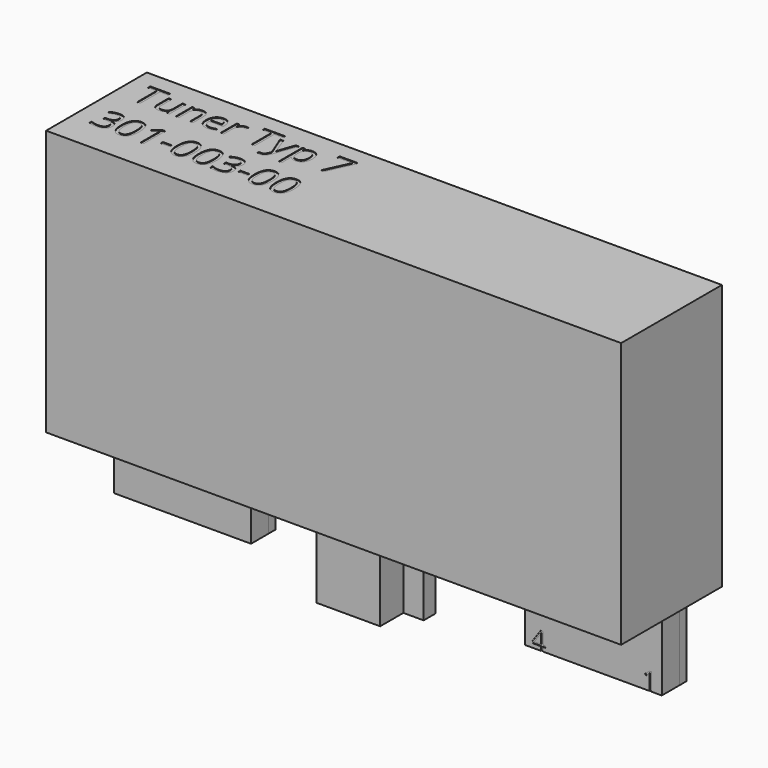
from build123d import *

# Parameters (mm, degrees)
F0_W          = 25
F0_H          = 14
F0_W_2        = 27
F1_DEPTH      = 1.6
F2_DEPTH      = 5
F3_DEPTH      = 18
F4_R          = 1.5
F5_DEPTH      = 14
F7_DEPTH      = 4
F9_TEXT_SIZE  = 6.9444444444
F10_DEPTH     = 0.1
F11_W         = 4
F11_H         = 2
F12_DEPTH     = 8
F13_W         = 4
F13_H         = 2
F14_DEPTH     = 8
F15_TEXT_SIZE = 4.5010312564
F16_DEPTH     = 0.1


# Not quite as in the source:
# - Text() gives the source's letters only with a copy of the font that has no kerning and outlines rounded to 1/6400 em; it was checked with that copy


with BuildPart() as f1:
    # F0 (on Front) → F1 (new body)
    with BuildSketch(Plane.XZ):
        Polygon((52.5, -24.25), (52.5, 24.25), (-52.5, 24.25), (-52.5, -24.25), (-50, -24.25), (-25, -24.25), (-10, -24.25), (9, -24.25), (23, -24.25), (50, -24.25), align=None)
        with Locations((-37.5, -31.25)):
            Rectangle(F0_W, F0_H)
        with Locations((36.5, -31.25)):
            Rectangle(F0_W_2, F0_H)
    extrude(amount=F1_DEPTH)

    # F0 (on Front) → F2 (join)
    with BuildSketch(Plane.XZ):
        Polygon((52.5, -24.25), (52.5, 24.25), (-52.5, 24.25), (-52.5, -24.25), (-50, -24.25), (-25, -24.25), (-10, -24.25), (9, -24.25), (23, -24.25), (50, -24.25), align=None)
    extrude(amount=-F2_DEPTH)

    # F0 (on Front) → F3 (join)
    with BuildSketch(Plane.XZ):
        Polygon((52.5, -24.25), (52.5, 24.25), (-52.5, 24.25), (-52.5, -24.25), (-50, -24.25), (-25, -24.25), (-10, -24.25), (9, -24.25), (23, -24.25), (50, -24.25), align=None)
    extrude(amount=F3_DEPTH)

    # F4 (on face) → F5 (join)
    with BuildSketch(Plane(origin=(0, 0, -24.25), x_dir=(1, 0, 0), z_dir=(0, 0, -1))):
        Polygon((-10, 8.7), (-10, 6), (9, 6), (9, 8.7), (5.3, 8.7), (5.3, 14), (-6.3, 14), (-6.3, 8.7), align=None)
        with Locations((-0.5, 10)):
            Circle(F4_R, mode=Mode.SUBTRACT)
    extrude(amount=F5_DEPTH)

    # F9 (on face) → F10 (cut)
    with BuildSketch(Plane.XY.offset(24.25)):
        with Locations((-49.5, -3)):
            Text('Tuner Typ 7', F9_TEXT_SIZE, font='Open Sans', text_align=(TextAlign.LEFT, TextAlign.BOTTOM))
        with Locations((-49.5, -12.4444444444)):
            Text('301-003-00', F9_TEXT_SIZE, font='Open Sans', text_align=(TextAlign.LEFT, TextAlign.BOTTOM))
    extrude(amount=-F10_DEPTH, mode=Mode.SUBTRACT)


with BuildPart() as f7:
    # F6 (on face) → F7 (new body)
    with BuildSketch(Plane.XZ.offset(1.6)):
        Polygon((-49, -24.25), (-50, -24.25), (-50, -38.25), (-25, -38.25), (-25, -24.25), (-26, -24.25), (-26, -26.25), (-49, -26.25), align=None)
    extrude(amount=F7_DEPTH)


with BuildPart() as f8_1:
    # F8: copy of F7
    add(f7.part.moved(Location((75, 0, 0))))

    # F13 (on face) → F14 (cut)
    with BuildSketch(Plane(origin=(0, 0, -38.25), x_dir=(1, 0, 0), z_dir=(0, 0, -1))):
        with Locations((32.5344918425, 3.6)):
            Rectangle(F13_W, F13_H)
        with Locations((37.5344918425, 3.6)):
            Rectangle(F13_W, F13_H)
        with Locations((42.5344918425, 3.6)):
            Rectangle(F13_W, F13_H)
        with Locations((47.5344918425, 3.6)):
            Rectangle(F13_W, F13_H)
        with Locations((27.5344918425, 3.6)):
            Rectangle(F13_W, F13_H)
    extrude(amount=-F14_DEPTH, mode=Mode.SUBTRACT)

    # F15 (on face) → F16 (cut)
    with BuildSketch(Plane.XZ.offset(5.6)):
        with Locations((46.5249736838, -38.25)):
            Text('1', F15_TEXT_SIZE, font='Open Sans', text_align=(TextAlign.LEFT, TextAlign.BOTTOM))
        with Locations((26.2596663088, -38.25)):
            Text('4', F15_TEXT_SIZE, font='Open Sans', text_align=(TextAlign.LEFT, TextAlign.BOTTOM))
    extrude(amount=-F16_DEPTH, mode=Mode.SUBTRACT)


with BuildPart() as f7_1:
    add(f7.part)

    # F11 (on face) → F12 (cut)
    with BuildSketch(Plane(origin=(0, 0, -38.25), x_dir=(1, 0, 0), z_dir=(0, 0, -1))):
        with Locations((-47.5, 3.6)):
            Rectangle(F11_W, F11_H)
        with Locations((-42.5, 3.6)):
            Rectangle(F11_W, F11_H)
        with Locations((-37.5, 3.6)):
            Rectangle(F11_W, F11_H)
        with Locations((-32.5, 3.6)):
            Rectangle(F11_W, F11_H)
        with Locations((-27.5, 3.6)):
            Rectangle(F11_W, F11_H)
    extrude(amount=-F12_DEPTH, mode=Mode.SUBTRACT)


solid = Compound([f1.part, f8_1.part, f7_1.part])
